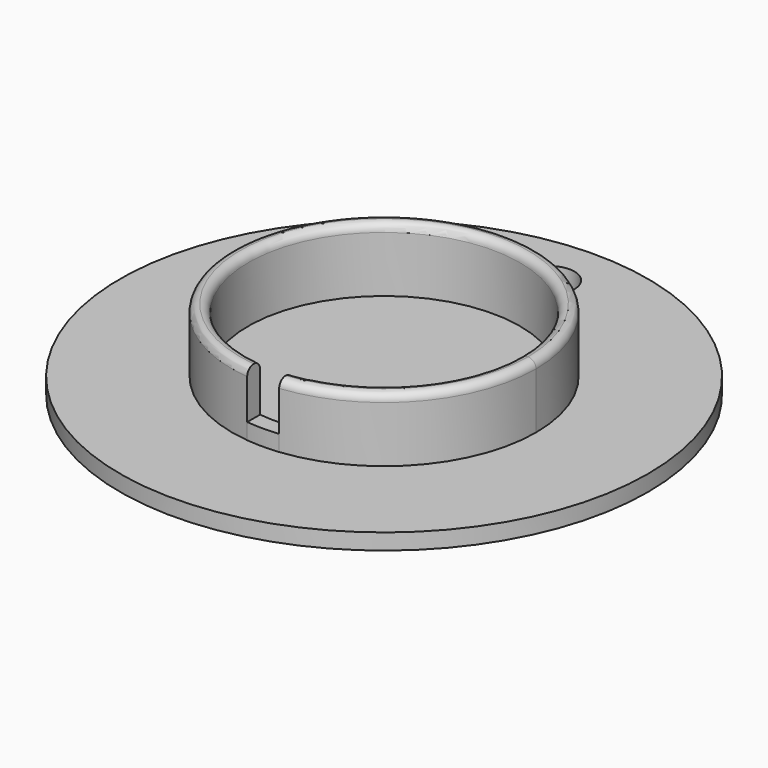
from build123d import *

# Parameters (mm, degrees)
F0_R     = 16.5
F0_R_2   = 1.5
F1_DEPTH = 1
F2_DEPTH = 5
F3_DEPTH = 2
F4_R     = 0.49999


# Not quite as in the source:
# - a fillet or chamfer is up to 0.001 mm smaller than in the source, because OpenCascade refuses the exact size


with BuildPart() as f1:
    # F0 (on Top) → F1 (new body)
    with BuildSketch(Plane.XY):
        Circle(F0_R)
        with BuildLine():
            ThreePointArc((-1, -9.4472218138), (-6.3541325136, 7.0622234459), (9.5, 0))
            ThreePointArc((9.5, 0), (7.0622234459, -6.3541325136), (1, -9.4472218138))
            ThreePointArc((1, -9.4472218138), (0, -9.5), (-1, -9.4472218138))
        make_face(mode=Mode.SUBTRACT)
        with Locations((0, 13)):
            Circle(F0_R_2, mode=Mode.SUBTRACT)
    extrude(amount=F1_DEPTH)


with BuildPart() as f1b:
    # F0 (on Top) → F1, piece 2 (new body)
    with BuildSketch(Plane.XY):
        with BuildLine():
            ThreePointArc((8.5, 0), (-5.6457948953, 6.3541325136), (-1, -8.4409715081))
            ThreePointArc((-1, -8.4409715081), (0, -8.5), (1, -8.4409715081))
            ThreePointArc((1, -8.4409715081), (6.3541325136, -5.6457948953), (8.5, 0))
        make_face()
    extrude(amount=F1_DEPTH)


with BuildPart() as f2:
    # F0 (on Top) → F2 (new body)
    with BuildSketch(Plane.XY):
        with BuildLine():
            ThreePointArc((1, -9.4472218138), (7.0622234459, -6.3541325136), (9.5, 0))
            ThreePointArc((9.5, 0), (-6.3541325136, 7.0622234459), (-1, -9.4472218138))
            Line((-1, -9.4472218138), (-1, -8.4409715081))
            ThreePointArc((-1, -8.4409715081), (-5.6457948953, 6.3541325136), (8.5, 0))
            ThreePointArc((8.5, 0), (6.3541325136, -5.6457948953), (1, -8.4409715081))
            Line((1, -8.4409715081), (1, -9.4472218138))
        make_face()
    extrude(amount=F2_DEPTH)

    # F4 (radius 0.5 in the source; OpenCascade refuses exactly that, so slightly less here)
    f4_edges = [f2.edges().sort_by_distance(p)[0] for p in [
        (0, 9.5, 5),
        (-5.645795, 6.354133, 5),
    ]]
    fillet(f4_edges, radius=F4_R)


with BuildPart() as f3:
    # F0 (on Top) → F3 (new body)
    with BuildSketch(Plane.XY):
        with BuildLine():
            Line((-1, -8.4409715081), (-1, -9.4472218138))
            ThreePointArc((-1, -9.4472218138), (0, -9.5), (1, -9.4472218138))
            Line((1, -9.4472218138), (1, -8.4409715081))
            ThreePointArc((1, -8.4409715081), (0, -8.5), (-1, -8.4409715081))
        make_face()
    extrude(amount=F3_DEPTH)


solid = Compound([f1.part, f1b.part, f2.part, f3.part])
